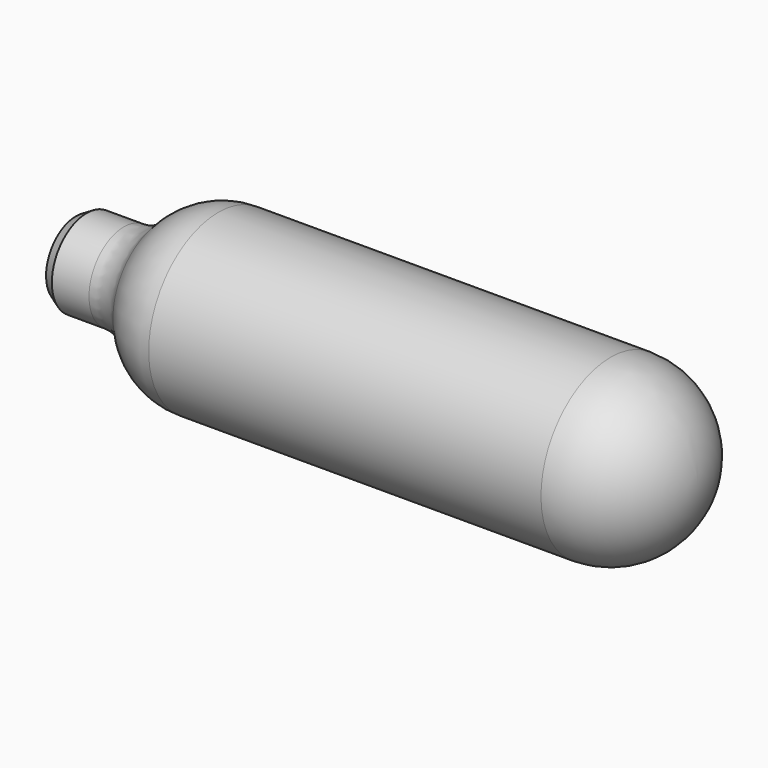
from build123d import *

# Parameters (mm, degrees)
F2_R = 8.89
F4_R = 5.08


# Not quite as in the source:
# - a fillet or chamfer that OpenCascade refuses, or shapes differently, is made with other operations: its cross-section is extruded or revolved along the edge and cut away or added


with BuildPart() as f1:
    # F0 (on Front) → F1 (revolve)
    with BuildSketch(Plane.XZ):
        Polygon((-19.955041249, 4.445), (-19.955041249, 0), (43.544958751, 0), (43.544958751, 8.89), (-12.335041249, 8.89), (-12.335041249, 4.445), align=None)
    revolve(axis=Axis((11.794958751, 0, 0), (1, 0, 0)))

    # F2
    f2_edges = [f1.edges().sort_by_distance(p)[0] for p in [
        (43.544959, 0, -8.89),
    ]]
    fillet(f2_edges, radius=F2_R)

    # F3: fillet of radius 7.62 on 1 edges, made by hand

    # F3_s1 → F3_t2 (revolve, cut)
    with BuildSketch(Plane.XZ):
        with BuildLine():
            ThreePointArc((-5.4080090562, 8.89), (-9.5232793997, 7.6831856359), (-12.335041249, 4.445))
            Line((-12.335041249, 4.445), (-12.335041249, 8.89))
            Line((-12.335041249, 8.89), (-5.4080090562, 8.89))
        make_face()
    revolve(axis=Axis((-12.335041249, 0, 0), (1, 0, 0)), mode=Mode.SUBTRACT)

    # F4
    f4_edges = [f1.edges().sort_by_distance(p)[0] for p in [
        (-12.335041, 0, -4.445),
    ]]
    fillet(f4_edges, radius=F4_R)

    # F5: chamfer of 0.635 x 1.0998522628 on 1 edges, made by hand

    # F5_s1 → F5_t2 (revolve, cut)
    with BuildSketch(Plane.XZ):
        Polygon((-18.8551889862, 4.445), (-19.955041249, 3.81), (-19.955041249, 4.445), align=None)
    revolve(axis=Axis((-19.955041249, 0, 0), (1, 0, 0)), mode=Mode.SUBTRACT)


solid = f1.part
